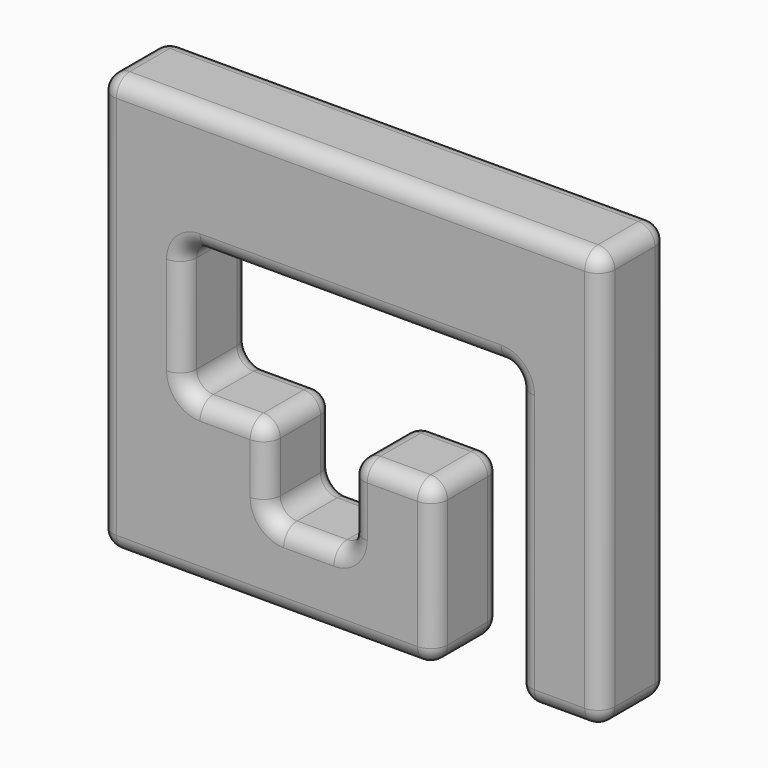
from build123d import *

# Parameters (mm, degrees)
F1_DEPTH = 12.7
F2_F1_R  = 5.08
F2_F2_R  = 5.08


with BuildPart() as f1:
    # F0 (on Front) → F1 (new body, symmetric)
    with BuildSketch(Plane.XZ):
        Polygon((152.4, 0), (0, 0), (0, -127), (101.6, -127), (101.6, -78.0620644748), (76.2, -78.0620644748), (76.2, -103.637776798), (50.8, -103.637776798), (50.8, -78.0620644748), (25.4, -78.0620644748), (25.4, -38.1), (127, -38.1), (127, -127), (152.4, -127), align=None)
    extrude(amount=F1_DEPTH, both=True)

    # F2: fillet of radius 5.08 on 40 edges, made by hand

    # F2_f1
    f2_f1_edges = [f1.edges().sort_by_distance(p)[0] for p in [
        (25.4, 0, -78.0620644748),
        (25.4, 0, -38.1),
        (127, 0, -38.1),
        (76.2, 0, -103.637776798),
        (50.8, 0, -103.637776798),
    ]]
    fillet(f2_f1_edges, radius=F2_F1_R)

    # F2_f2
    f2_f2_edges = [f1.edges().sort_by_distance(p)[0] for p in [
        (76.2, -12.7, 0),
        (76.2, 12.7, 0),
        (152.4, 0, 0),
        (0, 0, 0),
        (139.7, -12.7, -127),
        (152.4, 0, -127),
        (127, 0, -127),
        (139.7, 12.7, -127),
        (101.6, 0, -127),
        (50.8, -12.7, -127),
        (101.6, -12.7, -102.5310322374),
        (101.6, 12.7, -102.5310322374),
        (101.6, 0, -78.0620644748),
        (50.8, 12.7, -127),
        (0, 0, -127),
        (63.5, -12.7, -103.637776798),
        (76.2, -12.7, -88.3099206364),
        (50.8, -12.7, -88.3099206364),
        (50.8, 0, -78.0620644748),
        (50.8, 12.7, -88.3099206364),
        (63.5, 12.7, -103.637776798),
        (76.2, 0, -78.0620644748),
        (88.9, 12.7, -78.0620644748),
        (127, -12.7, -85.09),
        (127, 12.7, -85.09),
        (76.2, -12.7, -38.1),
        (25.4, -12.7, -58.0810322374),
        (40.64, -12.7, -78.0620644748),
        (0, -12.7, -63.5),
        (88.9, -12.7, -78.0620644748),
        (40.64, 12.7, -78.0620644748),
        (0, 12.7, -63.5),
        (25.4, 12.7, -58.0810322374),
        (152.4, -12.7, -63.5),
        (152.4, 12.7, -63.5),
        (26.8878975516, 12.7, -76.5741669232),
        (26.8878975516, 12.7, -39.5878975516),
        (26.8878975516, -12.7, -76.5741669232),
        (26.8878975516, -12.7, -39.5878975516),
        (125.5121024484, -12.7, -39.5878975516),
        (125.5121024484, 12.7, -39.5878975516),
        (74.7121024484, 12.7, -102.1498792464),
        (52.2878975516, 12.7, -102.1498792464),
        (52.2878975516, -12.7, -102.1498792464),
        (74.7121024484, -12.7, -102.1498792464),
    ]]
    fillet(f2_f2_edges, radius=F2_F2_R)


solid = f1.part
